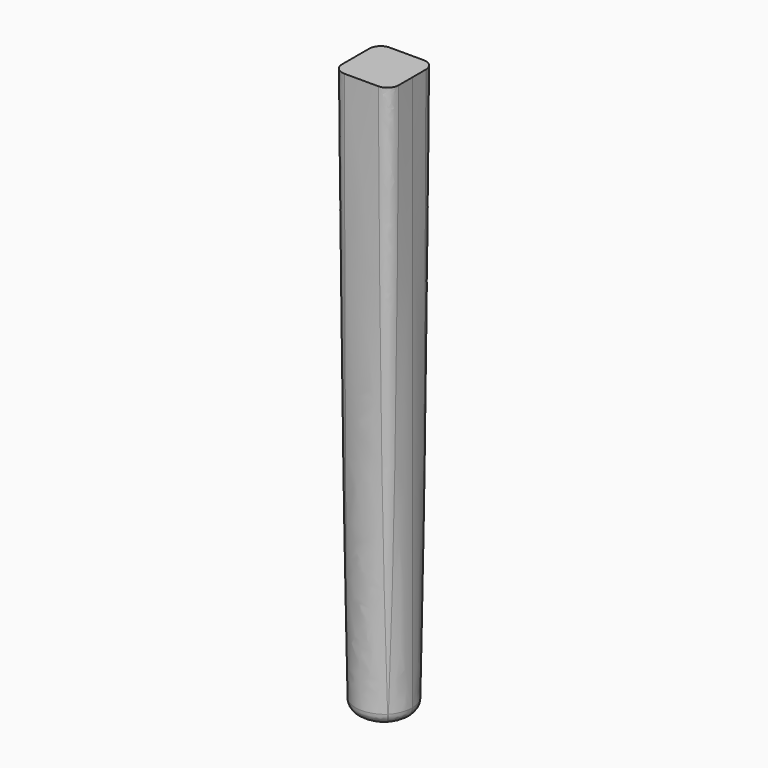
from build123d import *

# Parameters (mm, degrees)
F0_R    = 25
F2_W    = 50
F2_H    = 50
F4_F1_R = 10
F4_F2_R = 10
F4_F3_R = 10
F4_F4_R = 10
F4_F5_R = 10


with BuildPart() as f3:
    # F0 (on Top) → F3 section 0
    with BuildSketch(Plane.XY):
        Circle(F0_R)
    # F2 (on offset) → F3 section 1
    with BuildSketch(Plane.XY.offset(500)):
        Rectangle(F2_W, F2_H)
    loft()

    # F4: fillet of radius 10 on 9 edges, made by hand

    # F4_f1
    f4_f1_edges = [f3.edges().sort_by_distance(p)[0] for p in [
        (21.3388347648, 21.3388347648, 250),
    ]]
    fillet(f4_f1_edges, radius=F4_F1_R)

    # F4_f2
    f4_f2_edges = [f3.edges().sort_by_distance(p)[0] for p in [
        (-21.3388347648, 21.3388347648, 250),
    ]]
    fillet(f4_f2_edges, radius=F4_F2_R)

    # F4_f3
    f4_f3_edges = [f3.edges().sort_by_distance(p)[0] for p in [
        (-21.3388347648, -21.3388347648, 250),
    ]]
    fillet(f4_f3_edges, radius=F4_F3_R)

    # F4_f4
    f4_f4_edges = [f3.edges().sort_by_distance(p)[0] for p in [
        (21.3388347648, -21.3388347648, 250),
    ]]
    fillet(f4_f4_edges, radius=F4_F4_R)

    # F4_f5
    f4_f5_edges = [f3.edges().sort_by_distance(p)[0] for p in [
        (23.0969883128, 9.5670858091, 0),
        (0, 25, 0),
        (-25, 0, 0),
        (0, -25, 0),
        (23.0969883128, -9.5670858091, 0),
    ]]
    fillet(f4_f5_edges, radius=F4_F5_R)


solid = f3.part
